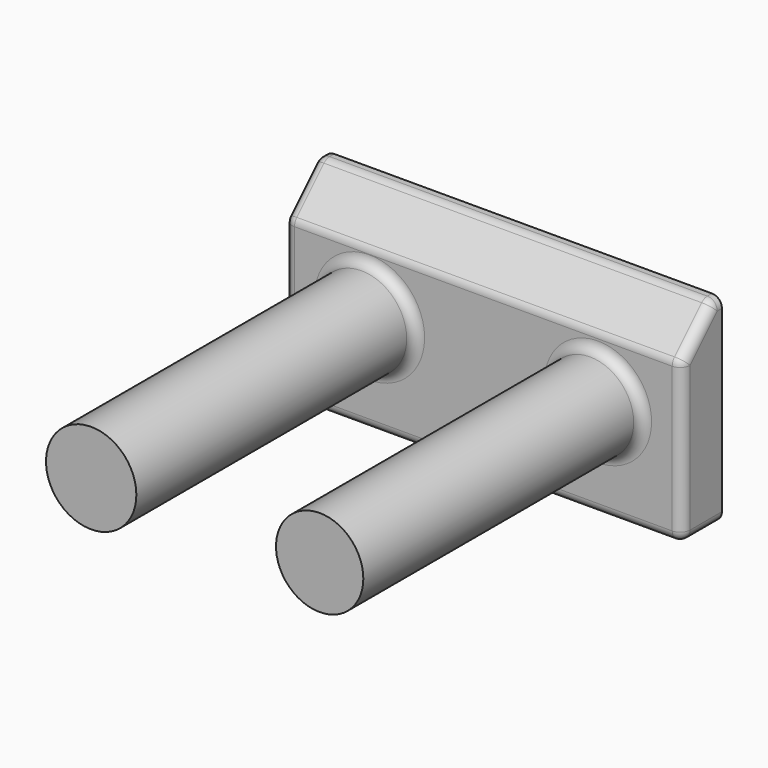
from build123d import *

# Parameters (mm, degrees)
F0_W     = 200
F0_H     = 100
F0_R     = 22.7241513298
F0_R_2   = 21.9586845422
F1_DEPTH = 25
F2_DEPTH = 200
F3_SIZE  = 20
F4_F1_R  = 5
F4_F2_R  = 5
F4_F3_R  = 5
F4_F4_R  = 5
F4_F5_R  = 5
F4_F6_R  = 5
F4_F7_R  = 5


# Not quite as in the source:
# - a feature of the source that left no trace in its solid (it failed there, or was rolled back) is left out


with BuildPart() as f1:
    # F0 (on Front) → F1 (new body)
    with BuildSketch(Plane.XZ):
        with Locations((-13.0278225988, -29.689514604)):
            Rectangle(F0_W, F0_H)
        with Locations((-70.3068226576, -29.689514604)):
            Circle(F0_R, mode=Mode.SUBTRACT)
        with Locations((44.6292310953, -29.689514604)):
            Circle(F0_R_2, mode=Mode.SUBTRACT)
    extrude(amount=F1_DEPTH)

    # F0 (on Front) → F2 (join)
    with BuildSketch(Plane.XZ):
        with Locations((44.6292310953, -29.689514604)):
            Circle(F0_R_2)
        with Locations((-70.3068226576, -29.689514604)):
            Circle(F0_R)
    extrude(amount=F2_DEPTH)

    # F3
    f3_edges = [f1.edges().sort_by_distance(p)[0] for p in [
        (-13.027823, -25, 20.310485),
    ]]
    chamfer(f3_edges, length=F3_SIZE)

    # F4: fillet of radius 5 on 11 edges, made by hand

    # F4_f1
    f4_f1_edges = [f1.edges().sort_by_distance(p)[0] for p in [
        (-13.0278225988, -5, 20.310485396),
    ]]
    fillet(f4_f1_edges, radius=F4_F1_R)

    # F4_f2
    f4_f2_edges = [f1.edges().sort_by_distance(p)[0] for p in [
        (-13.0278225988, -25, 0.310485396),
    ]]
    fillet(f4_f2_edges, radius=F4_F2_R)

    # F4_f3
    f4_f3_edges = [f1.edges().sort_by_distance(p)[0] for p in [
        (-13.0278225988, -25, -79.689514604),
    ]]
    fillet(f4_f3_edges, radius=F4_F3_R)

    # F4_f4
    f4_f4_edges = [f1.edges().sort_by_distance(p)[0] for p in [
        (-93.0309739873, -25, -29.689514604),
    ]]
    fillet(f4_f4_edges, radius=F4_F4_R)

    # F4_f5
    f4_f5_edges = [f1.edges().sort_by_distance(p)[0] for p in [
        (22.6705465531, -25, -29.689514604),
    ]]
    fillet(f4_f5_edges, radius=F4_F5_R)

    # F4_f6
    f4_f6_edges = [f1.edges().sort_by_distance(p)[0] for p in [
        (86.9721774012, -25, -38.2250485099),
    ]]
    fillet(f4_f6_edges, radius=F4_F6_R)

    # F4_f7
    f4_f7_edges = [f1.edges().sort_by_distance(p)[0] for p in [
        (-113.0278225988, -25, -38.2250485099),
    ]]
    fillet(f4_f7_edges, radius=F4_F7_R)


solid = f1.part
